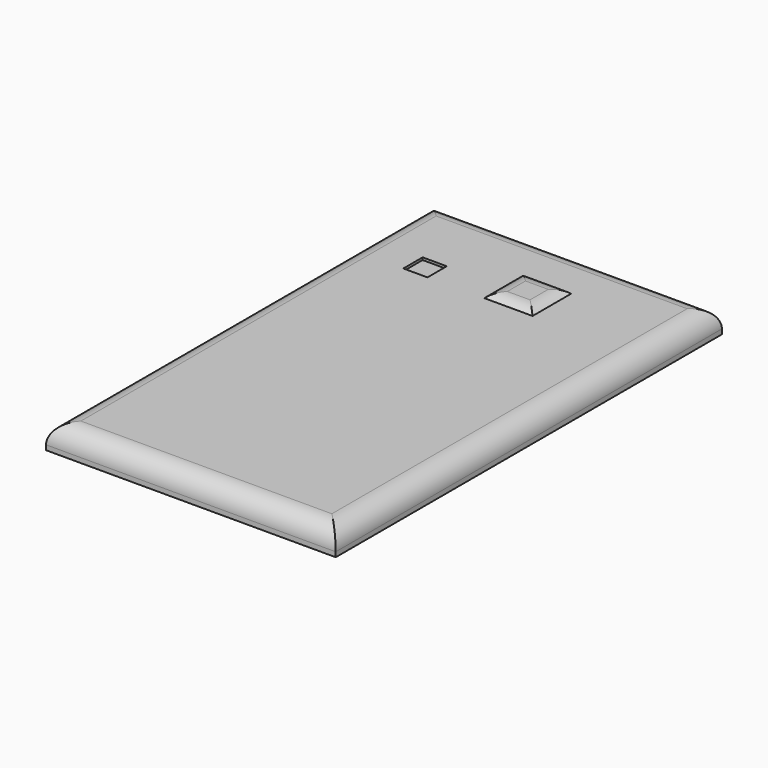
from build123d import *

# Parameters (mm, degrees)
F0_W        = 76.2
F0_H        = 127
F1_DEPTH    = 6.35
F2_W        = 12.7
F2_H        = 12.7
F3_DEPTH    = 1.27
F4_W        = 6.35
F4_H        = 6.35
F5_DEPTH    = 0.635
F6_T1_DEPTH = 29.5005208253
F6_T3_DEPTH = 29.5005208253
F6_T5_DEPTH = 152.4
F6_T7_DEPTH = 101.6


# Not quite as in the source:
# - a fillet or chamfer that OpenCascade refuses, or shapes differently, is made with other operations: its cross-section is extruded or revolved along the edge and cut away or added


with BuildPart() as f1:
    # F0 (on Top) → F1 (new body)
    with BuildSketch(Plane.XY):
        Rectangle(F0_W, F0_H)
    extrude(amount=F1_DEPTH)

    # F2 (on face) → F3 (join)
    with BuildSketch(Plane.XY.offset(6.35)):
        with Locations((3.8891917182, 42.4066188663)):
            Rectangle(F2_W, F2_H)
    extrude(amount=F3_DEPTH)

    # F4 (on face) → F5 (cut)
    with BuildSketch(Plane.XY.offset(6.35)):
        with Locations((-20.5224687852, 39.1501502216)):
            Rectangle(F4_W, F4_H)
    extrude(amount=-F5_DEPTH, mode=Mode.SUBTRACT)

    # F6: fillet of radius 5.08 on 8 edges, made by hand

    # F6_s2 → F6_t1 (cut)
    with BuildSketch(Plane.XZ.offset(-57.156879279)):
        with BuildLine():
            ThreePointArc((10.2391917182, 6.35), (8.6751387773, 7.2919048812), (6.8790875531, 7.62))
            Line((6.8790875531, 7.62), (10.2391917182, 7.62))
            Line((10.2391917182, 7.62), (10.2391917182, 6.35))
        make_face()
        with BuildLine():
            ThreePointArc((-2.4608082818, 6.35), (-0.896755341, 7.2919048812), (0.8992958832, 7.62))
            Line((0.8992958832, 7.62), (-2.4608082818, 7.62))
            Line((-2.4608082818, 7.62), (-2.4608082818, 6.35))
        make_face()
    extrude(amount=F6_T1_DEPTH, mode=Mode.SUBTRACT)

    # F6_s4 → F6_t3 (cut)
    with BuildSketch(Plane.YZ.offset(-10.8610686945)):
        with BuildLine():
            ThreePointArc((48.7566188663, 6.35), (47.1925659255, 7.2919048812), (45.3965147013, 7.62))
            Line((45.3965147013, 7.62), (48.7566188663, 7.62))
            Line((48.7566188663, 7.62), (48.7566188663, 6.35))
        make_face()
        with BuildLine():
            ThreePointArc((36.0566188663, 6.35), (37.6206718072, 7.2919048812), (39.4167230314, 7.62))
            Line((39.4167230314, 7.62), (36.0566188663, 7.62))
            Line((36.0566188663, 7.62), (36.0566188663, 6.35))
        make_face()
    extrude(amount=F6_T3_DEPTH, mode=Mode.SUBTRACT)

    # F6_s6 → F6_t5 (cut)
    with BuildSketch(Plane.XZ.offset(-76.2)):
        with BuildLine():
            ThreePointArc((38.1, 1.27), (36.6121024484, 4.8621024484), (33.02, 6.35))
            Line((33.02, 6.35), (38.1, 6.35))
            Line((38.1, 6.35), (38.1, 1.27))
        make_face()
        with BuildLine():
            ThreePointArc((-33.02, 6.35), (-36.6121024484, 4.8621024484), (-38.1, 1.27))
            Line((-38.1, 1.27), (-38.1, 6.35))
            Line((-38.1, 6.35), (-33.02, 6.35))
        make_face()
    extrude(amount=F6_T5_DEPTH, mode=Mode.SUBTRACT)

    # F6_s8 → F6_t7 (cut)
    with BuildSketch(Plane.YZ.offset(-50.8)):
        with BuildLine():
            ThreePointArc((-63.5, 1.27), (-62.0121024484, 4.8621024484), (-58.42, 6.35))
            Line((-58.42, 6.35), (-63.5, 6.35))
            Line((-63.5, 6.35), (-63.5, 1.27))
        make_face()
        with BuildLine():
            ThreePointArc((63.5, 1.27), (62.0121024484, 4.8621024484), (58.42, 6.35))
            Line((58.42, 6.35), (63.5, 6.35))
            Line((63.5, 6.35), (63.5, 1.27))
        make_face()
    extrude(amount=F6_T7_DEPTH, mode=Mode.SUBTRACT)


solid = f1.part
